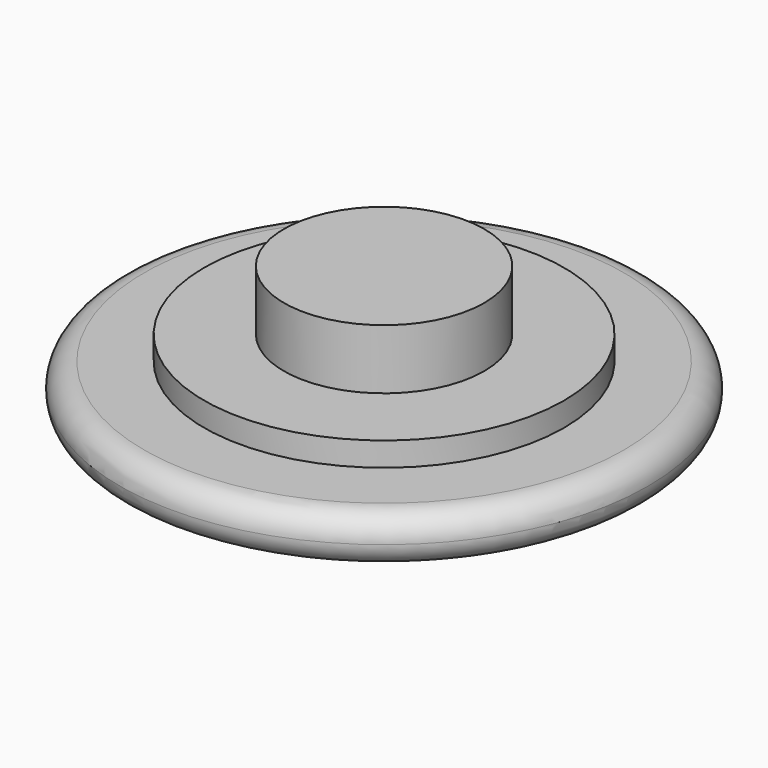
from build123d import *

# Parameters (mm, degrees)
F0_R         = 11
F0_R_2       = 7.5
F1_DEPTH     = 2
F0_R_3       = 4.175
F2_DEPTH     = 3
F3_DEPTH     = 5.5
F4_R         = 0.99999
F5_TEXT_SIZE = 5.0340107538
F6_DEPTH     = 1


# Not quite as in the source:
# - a fillet or chamfer is up to 0.001 mm smaller than in the source, because OpenCascade refuses the exact size
# - Text() gives the source's letters only with a copy of the font that has no kerning and outlines rounded to 1/6400 em; it was checked with that copy


with BuildPart() as f1:
    # F0 (on Top) → F1 (new body)
    with BuildSketch(Plane.XY):
        Circle(F0_R)
        Circle(F0_R_2, mode=Mode.SUBTRACT)
    extrude(amount=F1_DEPTH)

    # F0 (on Top) → F2 (join)
    with BuildSketch(Plane.XY):
        Circle(F0_R_2)
        Circle(F0_R_3, mode=Mode.SUBTRACT)
    extrude(amount=F2_DEPTH)

    # F0 (on Top) → F3 (join)
    with BuildSketch(Plane.XY):
        Circle(F0_R_3)
    extrude(amount=F3_DEPTH)

    # F4 (radius 1 in the source; OpenCascade refuses exactly that, so slightly less here)
    f4_edges = [f1.edges().sort_by_distance(p)[0] for p in [
        (-11, 0, 2),
        (-11, 0, 0),
    ]]
    fillet(f4_edges, radius=F4_R)

    # F5 (on face) → F6 (cut)
    with BuildSketch(Plane(origin=(0, 0, 0), x_dir=(1, 0, 0), z_dir=(0, 0, -1))):
        with Locations((-9.8363454226, -1.8017515722)):
            Text('Momma', F5_TEXT_SIZE, font='Open Sans', text_align=(TextAlign.LEFT, TextAlign.BOTTOM))
    extrude(amount=-F6_DEPTH, mode=Mode.SUBTRACT)


solid = f1.part
